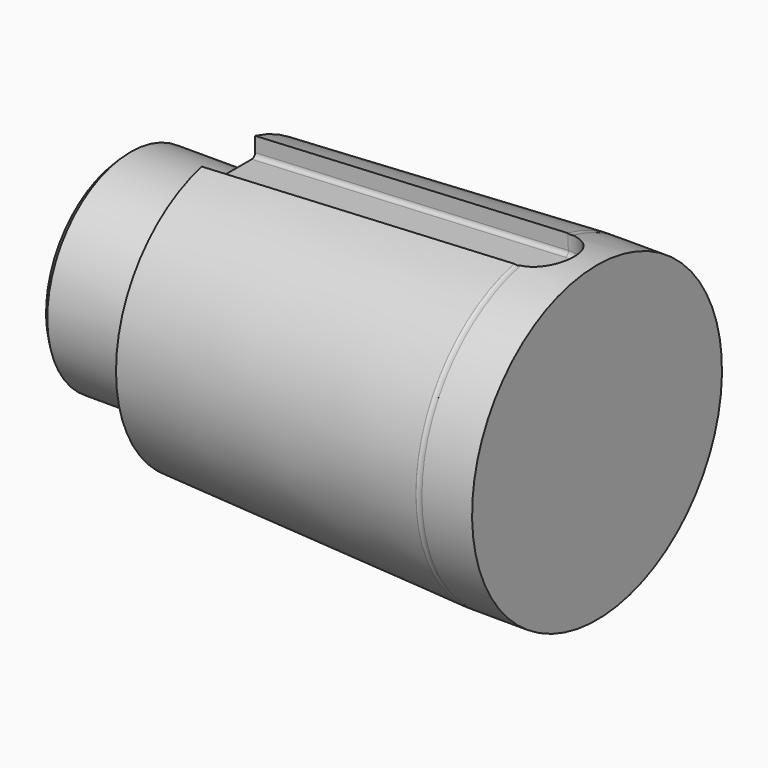
from build123d import *

# Parameters (mm, degrees)
F4_DEPTH = 11
F5_R     = 5
F7_SIZE  = 3
F8_R     = 2


# Not quite as in the source:
# - a pattern or mirror of a feature is missing from the dataset's text; its kind, count and spacing are read off the source's solid


with BuildPart() as f1:
    # F0 (on Front) → F1 (revolve)
    with BuildSketch(Plane.XZ):
        Polygon((0, 50), (0, 0), (227, 0), (227, 75), (200, 75), (50, 67.5), (50, 50), align=None)
    revolve(axis=Axis((113.5, 0, 0), (-1, 0, 0)))

    # F3 (on line) → F4 (cut)
    with BuildSketch(Plane(origin=(-3.2418952618, 0, 64.8379052369), x_dir=(0.9987523389, 0, 0.0499376169), z_dir=(-0.0499376169, 0, 0.9987523389))):
        with BuildLine():
            Line((0, 16), (0, -16))
            Line((0, -16), (203.4957890464, -16))
            ThreePointArc((203.4957890464, -16), (219.4957890464, 0), (203.4957890464, 16))
            Line((203.4957890464, 16), (0, 16))
        make_face()
    f4 = extrude(amount=-F4_DEPTH, mode=Mode.SUBTRACT)

    # F4_copies: F4 across plane
    add(f4.mirror(Plane(origin=(0, 0, -1e-06), x_dir=(-1, 0, 0), z_dir=(0, 0, -1))), mode=Mode.SUBTRACT)

    # F5 (on Front) → F6 (revolve, cut)
    with BuildSketch(Plane.XZ):
        with Locations((201.5, 79.8)):
            Circle(F5_R)
    revolve(axis=Axis((113.5, 0, 0), (-1, 0, 0)), mode=Mode.SUBTRACT)

    # F7
    f7_edges = [f1.edges().sort_by_distance(p)[0] for p in [
        (0, 0, -50),
    ]]
    chamfer(f7_edges, length=F7_SIZE)

    # F8
    f8_edges = [f1.edges().sort_by_distance(p)[0] for p in [
        (125.274657, 16, 60.249991),
        (216.529351, 0, 64.812726),
        (125.274657, -16, 60.249991),
        (125.274657, -16, -60.249993),
        (216.529351, 0, -64.812728),
        (125.274657, 16, -60.249993),
    ]]
    fillet(f8_edges, radius=F8_R)


solid = f1.part
